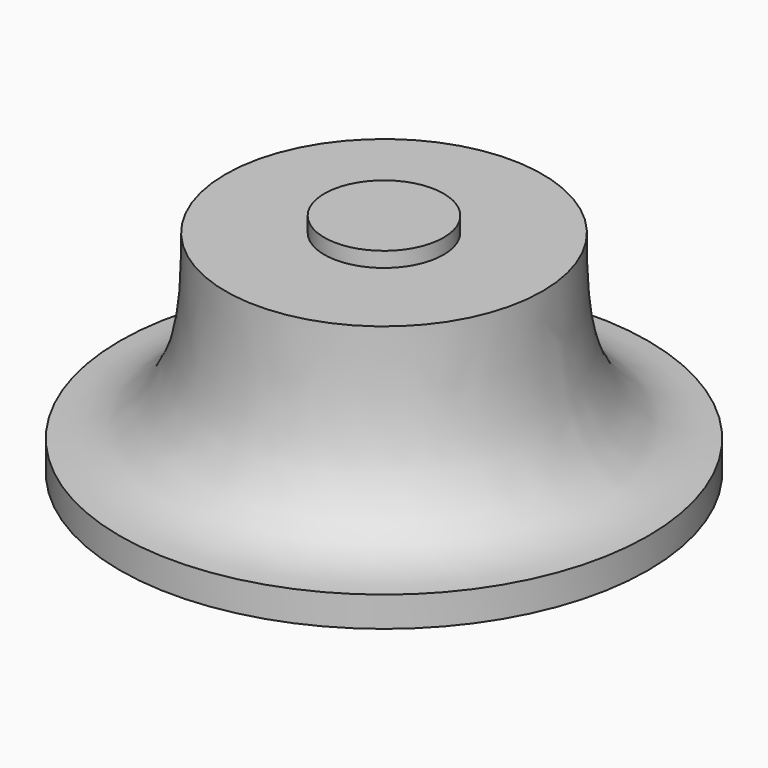
from build123d import *

# Parameters (mm, degrees)
F0_W = 2
F0_H = 1


# Not quite as in the source:
# - a feature names something its author has since deleted; it is built from what else it names


with BuildPart() as f1:
    # F0 (on Front) → F1 (revolve)
    with BuildSketch(Plane.XZ):
        with BuildLine():
            Line((10.5, 14), (3.95, 14))
            Line((3.95, 14), (2, 14))
            Line((2, 14), (2, 2))
            Line((2, 2), (17.5, 2))
            add(Edge.make_bspline(
                [(17.5, 2), (10.2541549131, 2), (10.5480328202, 10.096937418), (10.5, 14)],
                knots=[0, 0, 0, 0, 13.8924439894, 13.8924439894, 13.8924439894, 13.8924439894], degree=3))
        make_face()
        with BuildLine():
            Line((17.5, 0), (17.5, 2))
            Line((17.5, 2), (2, 2))
            Line((2, 2), (2, 1.9500468603))
            ThreePointArc((2, 1.9500468603), (7.3152696935, 1.3264671807), (12.5, 0))
            Line((12.5, 0), (17.5, 0))
        make_face()
        with Locations((1, 14.5)):
            Rectangle(F0_W, F0_H)
        Polygon((2, 14), (3.95, 14), (3.95, 15), (2.3, 15), (2, 15), align=None)
    revolve(axis=Axis((0, 0, 7), (0, 0, -1)))


solid = f1.part
